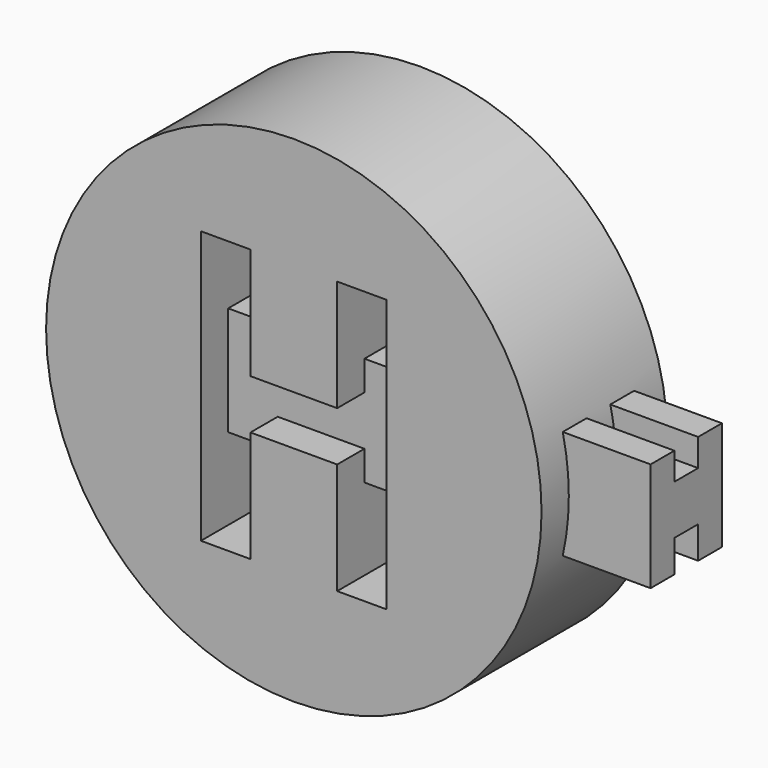
from build123d import *

# Parameters (mm, degrees)
F0_R     = 10
F1_DEPTH = 6.35
F4_DEPTH = 23
F5_DEPTH = 3
F6_DEPTH = 25


# Not quite as in the source:
# - a feature names something its author has since deleted; it is built from what else it names


with BuildPart() as f1:
    # F0 (on Front) → F1 (new body)
    with BuildSketch(Plane.XZ):
        Circle(F0_R)
        Polygon((-3.75, -5.5), (-3.75, -1), (-3.75, 1), (-3.75, 5.5), (-1.75, 5.5), (-1.75, 1), (1.75, 1), (1.75, 5.5), (3.75, 5.5), (3.75, 1), (3.75, -1), (3.75, -5.5), (1.75, -5.5), (1.75, -1), (-1.75, -1), (-1.75, -5.5), align=None, mode=Mode.SUBTRACT)
    extrude(amount=F1_DEPTH)

    # F3 (on offset) → F4 (join)
    with BuildSketch(Plane.YZ.offset(-9.7)):
        Polygon((-1.375, -2.2), (-1.375, 0), (-1.375, 2.2), (-2.575, 2.2), (-2.575, 1.0935393064), (-3.775, 1.0935393064), (-3.775, 2.2), (-4.975, 2.2), (-4.975, -2.2), (-3.775, -2.2), (-3.775, -0.9002136735), (-2.575, -0.9002136735), (-2.575, -2.2), align=None)
    extrude(amount=F4_DEPTH)

    # F3 (on offset) → F5 (cut)
    with BuildSketch(Plane.YZ.offset(-9.7)):
        Polygon((-1.375, -2.2), (-1.375, 0), (-1.375, 2.2), (-2.575, 2.2), (-2.575, 1.0935393064), (-3.775, 1.0935393064), (-3.775, 2.2), (-4.975, 2.2), (-4.975, -2.2), (-3.775, -2.2), (-3.775, -0.9002136735), (-2.575, -0.9002136735), (-2.575, -2.2), align=None)
    extrude(amount=F5_DEPTH, mode=Mode.SUBTRACT)

    # F3 (on offset) → F6 (cut)
    with BuildSketch(Plane.YZ.offset(-9.7)):
        Polygon((-1.375, -2.2), (-1.375, 0), (-1.375, 2.2), (-2.575, 2.2), (-2.575, 1.0935393064), (-3.775, 1.0935393064), (-3.775, 2.2), (-4.975, 2.2), (-4.975, -2.2), (-3.775, -2.2), (-3.775, -0.9002136735), (-2.575, -0.9002136735), (-2.575, -2.2), align=None)
    extrude(amount=-F6_DEPTH, mode=Mode.SUBTRACT)


solid = f1.part
